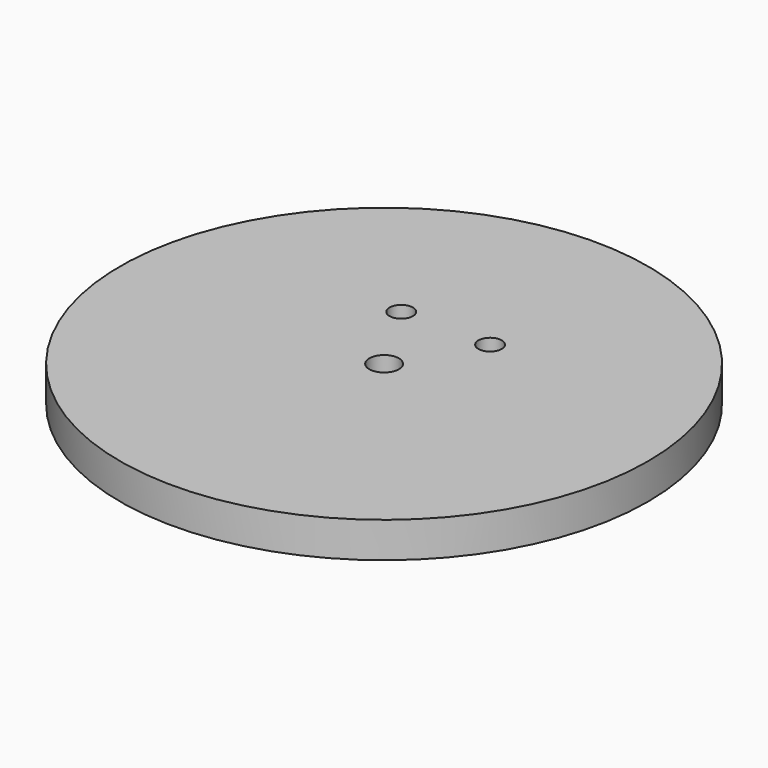
from build123d import *

# Parameters (mm, degrees)
F0_R     = 148.5
F0_R_2   = 6.5786
F0_R_3   = 8.3312
F1_DEPTH = 20
F2_R     = 146.5
F2_R_2   = 142
F3_DEPTH = 5


# Not quite as in the source:
# - a feature names something its author has since deleted; it is built from what else it names


with BuildPart() as f1:
    # F0 (on Top) → F1 (new body)
    with BuildSketch(Plane.XY):
        Circle(F0_R)
        with Locations((-25, 43.3012701892)):
            Circle(F0_R_2, mode=Mode.SUBTRACT)
        Circle(F0_R_3, mode=Mode.SUBTRACT)
        with Locations((25, 43.3012701892)):
            Circle(F0_R_2, mode=Mode.SUBTRACT)
    extrude(amount=F1_DEPTH)

    # F2 (on face) → F3 (cut)
    with BuildSketch(Plane.XY):
        Circle(F2_R)
        Circle(F2_R_2, mode=Mode.SUBTRACT)
    extrude(amount=F3_DEPTH, mode=Mode.SUBTRACT)


solid = f1.part
